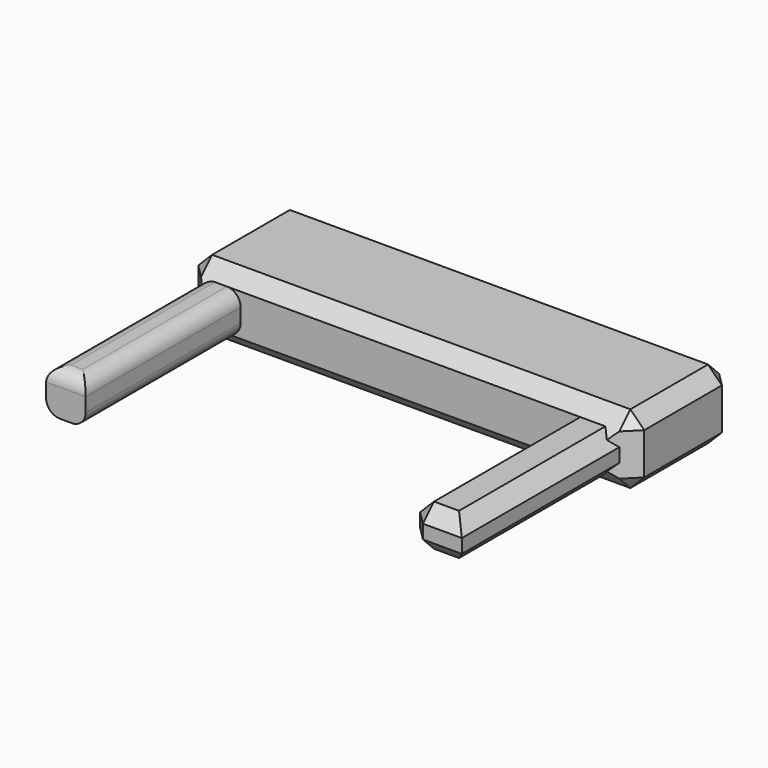
from build123d import *

# Parameters (mm, degrees)
F0_W         = 163.3519083261
F0_H         = 45.7251667976
F1_DEPTH     = 25.4
F2_SIZE      = 5.08
F3_W         = 14.5046669376
F3_H         = 15.24
F4_DEPTH     = 70.9391236305
F5_W         = 19.3313653898
F5_H         = 15.24
F6_DEPTH     = 72.0867142081
F7_T1_DEPTH  = 39.9046669376
F7_T6_DEPTH  = 96.3391236305
F7_T12_DEPTH = 96.3391236305
F7_T18_DEPTH = 96.3391236305
F7_T24_DEPTH = 83.6391236305
F7_T29_DEPTH = 83.6391236305
F7_T34_DEPTH = 83.6391236305
F7_T39_DEPTH = 83.6391236305
F7_T44_DEPTH = 96.3391236305
F7_T50_DEPTH = 96.3391236305
F7_T56_DEPTH = 96.3391236305
F8_T1_DEPTH  = 6.4524666085
F8_T3_DEPTH  = 6.4524666085
F8_T5_DEPTH  = 85.150863787
F8_T7_DEPTH  = 45.4596645476
F8_T9_DEPTH  = 41.3682991577
F8_T14_DEPTH = 98.2150133659
F8_T19_DEPTH = 98.2150133659
F8_T24_DEPTH = 98.2150133659
F8_T29_DEPTH = 98.2150133659


# Not quite as in the source:
# - a fillet or chamfer that OpenCascade refuses, or shapes differently, is made with other operations: its cross-section is extruded or revolved along the edge and cut away or added


with BuildPart() as f1:
    # F0 (on Top) → F1 (new body)
    with BuildSketch(Plane.XY):
        with Locations((39.7221744061, 22.8625833988)):
            Rectangle(F0_W, F0_H)
    extrude(amount=F1_DEPTH)

    # F2
    f2_edges = [f1.edges().sort_by_distance(p)[0] for p in [
        (121.398129, 22.862583, 25.4),
        (121.398129, 22.862583, 0),
        (39.722174, 0, 0),
        (121.398129, 0, 12.7),
        (121.398129, 45.725167, 12.7),
        (39.722174, 45.725167, 0),
        (39.722174, 45.725167, 25.4),
        (-41.95378, 22.862583, 25.4),
        (-41.95378, 0, 12.7),
        (-41.95378, 22.862583, 0),
        (-41.95378, 45.725167, 12.7),
        (39.722174, 0, 25.4),
    ]]
    chamfer(f2_edges, length=F2_SIZE)

    # F3 (on face) → F4 (join)
    with BuildSketch(Plane.XZ):
        with Locations((-29.6214462882, 12.7)):
            Rectangle(F3_W, F3_H)
    extrude(amount=F4_DEPTH)

    # F5 (on face) → F6 (join)
    with BuildSketch(Plane.XZ):
        with Locations((106.6524458742, 12.7)):
            Rectangle(F5_W, F5_H)
    extrude(amount=F6_DEPTH)

    # F7: fillet of radius 5.08 on 5 edges, made by hand

    # F7_s2 → F7_t1 (cut)
    with BuildSketch(Plane.YZ.offset(-49.573779757)):
        with BuildLine():
            ThreePointArc((-65.8591236305, 20.32), (-69.451226079, 18.8321024484), (-70.9391236305, 15.24))
            Line((-70.9391236305, 15.24), (-70.9391236305, 20.32))
            Line((-70.9391236305, 20.32), (-65.8591236305, 20.32))
        make_face()
    extrude(amount=F7_T1_DEPTH, mode=Mode.SUBTRACT)


with BuildPart() as f7_tool4:
    # F7_s5 → F7_t6 (new body)
    with BuildSketch(Plane.XZ.offset(-12.7)):
        with BuildLine():
            ThreePointArc((-36.873779757, 15.24), (-35.3858822055, 18.8321024484), (-31.793779757, 20.32))
            Line((-31.793779757, 20.32), (-36.873779757, 20.32))
            Line((-36.873779757, 20.32), (-36.873779757, 15.24))
        make_face()
    extrude(amount=F7_T6_DEPTH)

    split(bisect_by=Plane(origin=(-18.4368898785, -18.4368898785, 0), x_dir=(0, 0, 1), z_dir=(0.7071067812, 0.7071067812, 0)), keep=Keep.TOP)

    split(bisect_by=Plane(origin=(0, -10.16, 10.16), x_dir=(1, 0, 0), z_dir=(0, -0.7071067812, 0.7071067812)), keep=Keep.TOP)


with BuildPart() as f1_1:
    add(f1.part)

    # F7_t3: cut F7_tool4
    add(f7_tool4.part, mode=Mode.SUBTRACT)


with BuildPart() as f7_tool10:
    # F7_s11 → F7_t12 (new body)
    with BuildSketch(Plane.XZ.offset(-12.7)):
        with BuildLine():
            ThreePointArc((-36.873779757, 15.24), (-35.3858822055, 18.8321024484), (-31.793779757, 20.32))
            Line((-31.793779757, 20.32), (-36.873779757, 20.32))
            Line((-36.873779757, 20.32), (-36.873779757, 15.24))
        make_face()
    extrude(amount=F7_T12_DEPTH)

    split(bisect_by=Plane(origin=(-18.4368898785, -18.4368898785, 0), x_dir=(0, 0, 1), z_dir=(-0.7071067812, -0.7071067812, 0)), keep=Keep.TOP)

    split(bisect_by=Plane(origin=(0, -10.16, 10.16), x_dir=(1, 0, 0), z_dir=(0, 0.7071067812, -0.7071067812)), keep=Keep.TOP)


with BuildPart() as f1_2:
    add(f1_1.part)

    # F7_t9: cut F7_tool10
    add(f7_tool10.part, mode=Mode.SUBTRACT)


with BuildPart() as f7_tool16:
    # F7_s17 → F7_t18 (new body)
    with BuildSketch(Plane.XZ.offset(-12.7)):
        with BuildLine():
            ThreePointArc((-36.873779757, 15.24), (-35.3858822055, 18.8321024484), (-31.793779757, 20.32))
            Line((-31.793779757, 20.32), (-36.873779757, 20.32))
            Line((-36.873779757, 20.32), (-36.873779757, 15.24))
        make_face()
    extrude(amount=F7_T18_DEPTH)

    split(bisect_by=Plane(origin=(-18.4368898785, -18.4368898785, 0), x_dir=(0, 0, 1), z_dir=(-0.7071067812, -0.7071067812, 0)), keep=Keep.TOP)

    split(bisect_by=Plane(origin=(0, -10.16, 10.16), x_dir=(1, 0, 0), z_dir=(0, -0.7071067812, 0.7071067812)), keep=Keep.TOP)


with BuildPart() as f1_3:
    add(f1_2.part)

    # F7_t15: cut F7_tool16
    add(f7_tool16.part, mode=Mode.SUBTRACT)


with BuildPart() as f7_tool22:
    # F7_s23 → F7_t24 (new body)
    with BuildSketch(Plane.XZ):
        with BuildLine():
            ThreePointArc((-27.4491128194, 5.08), (-23.857010371, 6.5678975516), (-22.3691128194, 10.16))
            Line((-22.3691128194, 10.16), (-22.3691128194, 5.08))
            Line((-22.3691128194, 5.08), (-27.4491128194, 5.08))
        make_face()
    extrude(amount=F7_T24_DEPTH)

    split(bisect_by=Plane(origin=(0, 2.54, 2.54), x_dir=(1, 0, 0), z_dir=(0, 0.7071067812, 0.7071067812)), keep=Keep.TOP)


with BuildPart() as f1_4:
    add(f1_3.part)

    # F7_t21: cut F7_tool22
    add(f7_tool22.part, mode=Mode.SUBTRACT)


with BuildPart() as f7_tool27:
    # F7_s28 → F7_t29 (new body)
    with BuildSketch(Plane.XZ):
        with BuildLine():
            ThreePointArc((-27.4491128194, 5.08), (-23.857010371, 6.5678975516), (-22.3691128194, 10.16))
            Line((-22.3691128194, 10.16), (-22.3691128194, 5.08))
            Line((-22.3691128194, 5.08), (-27.4491128194, 5.08))
        make_face()
    extrude(amount=F7_T29_DEPTH)

    split(bisect_by=Plane(origin=(0, 2.54, 2.54), x_dir=(1, 0, 0), z_dir=(0, -0.7071067812, -0.7071067812)), keep=Keep.TOP)


with BuildPart() as f1_5:
    add(f1_4.part)

    # F7_t26: cut F7_tool27
    add(f7_tool27.part, mode=Mode.SUBTRACT)


with BuildPart() as f7_tool32:
    # F7_s33 → F7_t34 (new body)
    with BuildSketch(Plane.XZ):
        with BuildLine():
            ThreePointArc((-27.4491128194, 20.32), (-23.857010371, 18.8321024484), (-22.3691128194, 15.24))
            Line((-22.3691128194, 15.24), (-22.3691128194, 20.32))
            Line((-22.3691128194, 20.32), (-27.4491128194, 20.32))
        make_face()
    extrude(amount=F7_T34_DEPTH)

    split(bisect_by=Plane(origin=(0, -10.16, 10.16), x_dir=(1, 0, 0), z_dir=(0, 0.7071067812, -0.7071067812)), keep=Keep.TOP)


with BuildPart() as f1_6:
    add(f1_5.part)

    # F7_t31: cut F7_tool32
    add(f7_tool32.part, mode=Mode.SUBTRACT)


with BuildPart() as f7_tool37:
    # F7_s38 → F7_t39 (new body)
    with BuildSketch(Plane.XZ):
        with BuildLine():
            ThreePointArc((-27.4491128194, 20.32), (-23.857010371, 18.8321024484), (-22.3691128194, 15.24))
            Line((-22.3691128194, 15.24), (-22.3691128194, 20.32))
            Line((-22.3691128194, 20.32), (-27.4491128194, 20.32))
        make_face()
    extrude(amount=F7_T39_DEPTH)

    split(bisect_by=Plane(origin=(0, -10.16, 10.16), x_dir=(1, 0, 0), z_dir=(0, -0.7071067812, 0.7071067812)), keep=Keep.TOP)


with BuildPart() as f1_7:
    add(f1_6.part)

    # F7_t36: cut F7_tool37
    add(f7_tool37.part, mode=Mode.SUBTRACT)


with BuildPart() as f7_tool42:
    # F7_s43 → F7_t44 (new body)
    with BuildSketch(Plane.XZ.offset(-12.7)):
        with BuildLine():
            ThreePointArc((-36.873779757, 10.16), (-35.3858822055, 6.5678975516), (-31.793779757, 5.08))
            Line((-31.793779757, 5.08), (-36.873779757, 5.08))
            Line((-36.873779757, 5.08), (-36.873779757, 10.16))
        make_face()
    extrude(amount=F7_T44_DEPTH)

    split(bisect_by=Plane(origin=(-18.4368898785, -18.4368898785, 0), x_dir=(0, 0, 1), z_dir=(0.7071067812, 0.7071067812, 0)), keep=Keep.TOP)

    split(bisect_by=Plane(origin=(0, 2.54, 2.54), x_dir=(1, 0, 0), z_dir=(0, -0.7071067812, -0.7071067812)), keep=Keep.TOP)


with BuildPart() as f1_8:
    add(f1_7.part)

    # F7_t41: cut F7_tool42
    add(f7_tool42.part, mode=Mode.SUBTRACT)


with BuildPart() as f7_tool48:
    # F7_s49 → F7_t50 (new body)
    with BuildSketch(Plane.XZ.offset(-12.7)):
        with BuildLine():
            ThreePointArc((-36.873779757, 10.16), (-35.3858822055, 6.5678975516), (-31.793779757, 5.08))
            Line((-31.793779757, 5.08), (-36.873779757, 5.08))
            Line((-36.873779757, 5.08), (-36.873779757, 10.16))
        make_face()
    extrude(amount=F7_T50_DEPTH)

    split(bisect_by=Plane(origin=(-18.4368898785, -18.4368898785, 0), x_dir=(0, 0, 1), z_dir=(-0.7071067812, -0.7071067812, 0)), keep=Keep.TOP)

    split(bisect_by=Plane(origin=(0, 2.54, 2.54), x_dir=(1, 0, 0), z_dir=(0, 0.7071067812, 0.7071067812)), keep=Keep.TOP)


with BuildPart() as f1_9:
    add(f1_8.part)

    # F7_t47: cut F7_tool48
    add(f7_tool48.part, mode=Mode.SUBTRACT)


with BuildPart() as f7_tool54:
    # F7_s55 → F7_t56 (new body)
    with BuildSketch(Plane.XZ.offset(-12.7)):
        with BuildLine():
            ThreePointArc((-36.873779757, 10.16), (-35.3858822055, 6.5678975516), (-31.793779757, 5.08))
            Line((-31.793779757, 5.08), (-36.873779757, 5.08))
            Line((-36.873779757, 5.08), (-36.873779757, 10.16))
        make_face()
    extrude(amount=F7_T56_DEPTH)

    split(bisect_by=Plane(origin=(-18.4368898785, -18.4368898785, 0), x_dir=(0, 0, 1), z_dir=(-0.7071067812, -0.7071067812, 0)), keep=Keep.TOP)

    split(bisect_by=Plane(origin=(0, 2.54, 2.54), x_dir=(1, 0, 0), z_dir=(0, -0.7071067812, -0.7071067812)), keep=Keep.TOP)


with BuildPart() as f1_10:
    add(f1_9.part)

    # F7_t53: cut F7_tool54
    add(f7_tool54.part, mode=Mode.SUBTRACT)

    # F8: chamfer of 5.08 on 7 edges, made by hand

    # F8_s2 → F8_t1 (cut)
    with BuildSketch(Plane(origin=(4.9133496571, 4.9133496571, -4.9133496571), x_dir=(0.7071067812, -0.7071067812, 0), z_dir=(-0.5773502692, -0.5773502692, 0.5773502692))):
        Polygon((119.5530023794, 30.9044155805), (123.1451048279, 24.6827116338), (115.960899931, 24.6827116338), align=None)
    extrude(amount=F8_T1_DEPTH, mode=Mode.SUBTRACT)

    # F8_s4 → F8_t3 (cut)
    with BuildSketch(Plane(origin=(13.3800163237, 13.3800163237, 13.3800163237), x_dir=(0.7071067812, -0.7071067812, 0), z_dir=(-0.5773502692, -0.5773502692, -0.5773502692))):
        Polygon((119.5530023794, -10.1654024249), (123.1451048279, -3.9436984783), (115.960899931, -3.9436984783), align=None)
    extrude(amount=F8_T3_DEPTH, mode=Mode.SUBTRACT)

    # F8_s6 → F8_t5 (cut)
    with BuildSketch(Plane.XZ):
        Polygon((96.9867631793, 15.24), (102.0667631793, 20.32), (96.9867631793, 20.32), align=None)
        Polygon((96.9867631793, 10.16), (102.0667631793, 5.08), (96.9867631793, 5.08), align=None)
    extrude(amount=F8_T5_DEPTH, mode=Mode.SUBTRACT)

    # F8_s8 → F8_t7 (cut)
    with BuildSketch(Plane.YZ.offset(83.9226136004)):
        Polygon((-72.0867142081, 15.24), (-67.0067142081, 20.32), (-72.0867142081, 20.32), align=None)
        Polygon((-72.0867142081, 10.16), (-67.0067142081, 5.08), (-72.0867142081, 5.08), align=None)
    extrude(amount=F8_T7_DEPTH, mode=Mode.SUBTRACT)

    # F8_s10 → F8_t9 (cut)
    with BuildSketch(Plane.XY.offset(-7.9841495789)):
        Polygon((102.0667631793, -72.0867142081), (96.9867631793, -67.0067142081), (96.9867631793, -72.0867142081), align=None)
    extrude(amount=F8_T9_DEPTH, mode=Mode.SUBTRACT)


with BuildPart() as f8_tool12:
    # F8_s13 → F8_t14 (new body)
    with BuildSketch(Plane.XZ.offset(-13.0641495789)):
        Polygon((116.3181285691, 15.24), (111.2381285691, 20.32), (116.3181285691, 20.32), align=None)
    extrude(amount=F8_T14_DEPTH)

    split(bisect_by=Plane(origin=(0, -10.16, 10.16), x_dir=(1, 0, 0), z_dir=(0, -0.7071067812, 0.7071067812)), keep=Keep.TOP)


with BuildPart() as f1_11:
    add(f1_10.part)

    # F8_t11: cut F8_tool12
    add(f8_tool12.part, mode=Mode.SUBTRACT)


with BuildPart() as f8_tool17:
    # F8_s18 → F8_t19 (new body)
    with BuildSketch(Plane.XZ.offset(-13.0641495789)):
        Polygon((116.3181285691, 15.24), (111.2381285691, 20.32), (116.3181285691, 20.32), align=None)
    extrude(amount=F8_T19_DEPTH)

    split(bisect_by=Plane(origin=(58.1590642846, -58.1590642846, 0), x_dir=(0, 0, 1), z_dir=(0.7071067812, -0.7071067812, 0)), keep=Keep.TOP)


with BuildPart() as f1_12:
    add(f1_11.part)

    # F8_t16: cut F8_tool17
    add(f8_tool17.part, mode=Mode.SUBTRACT)


with BuildPart() as f8_tool22:
    # F8_s23 → F8_t24 (new body)
    with BuildSketch(Plane.XZ.offset(-13.0641495789)):
        Polygon((116.3181285691, 10.16), (111.2381285691, 5.08), (116.3181285691, 5.08), align=None)
    extrude(amount=F8_T24_DEPTH)

    split(bisect_by=Plane(origin=(0, 2.54, 2.54), x_dir=(1, 0, 0), z_dir=(0, -0.7071067812, -0.7071067812)), keep=Keep.TOP)


with BuildPart() as f1_13:
    add(f1_12.part)

    # F8_t21: cut F8_tool22
    add(f8_tool22.part, mode=Mode.SUBTRACT)


with BuildPart() as f8_tool27:
    # F8_s28 → F8_t29 (new body)
    with BuildSketch(Plane.XZ.offset(-13.0641495789)):
        Polygon((116.3181285691, 10.16), (111.2381285691, 5.08), (116.3181285691, 5.08), align=None)
    extrude(amount=F8_T29_DEPTH)

    split(bisect_by=Plane(origin=(58.1590642846, -58.1590642846, 0), x_dir=(0, 0, 1), z_dir=(0.7071067812, -0.7071067812, 0)), keep=Keep.TOP)


with BuildPart() as f1_14:
    add(f1_13.part)

    # F8_t26: cut F8_tool27
    add(f8_tool27.part, mode=Mode.SUBTRACT)


solid = f1_14.part
